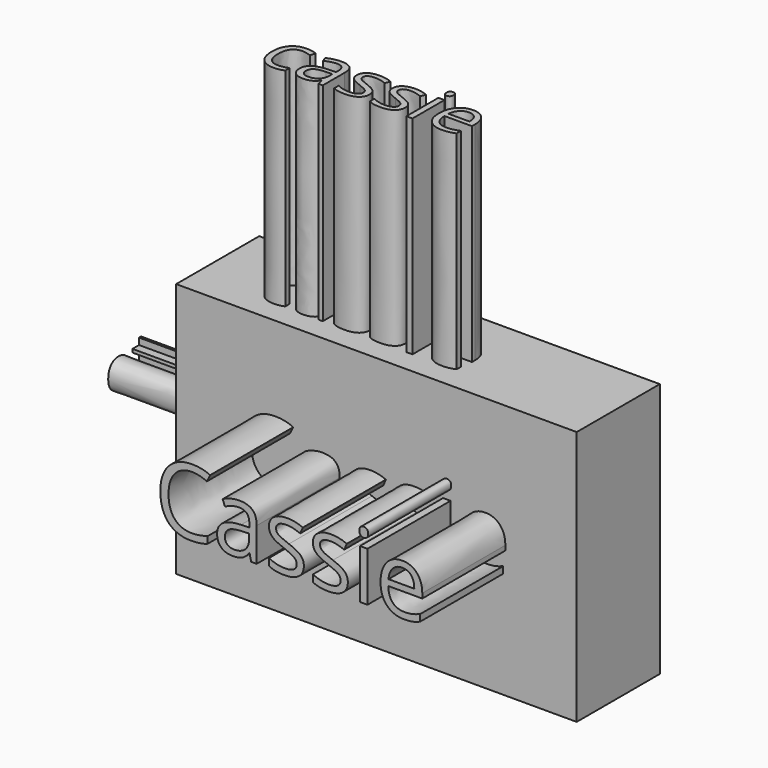
from build123d import *

# Parameters (mm, degrees)
F0_W         = 97.9832615703
F0_H         = 62.4232683331
F1_DEPTH     = 25.4
F2_TEXT_SIZE = 22.5471012527
F3_DEPTH     = 25.4
F4_TEXT_SIZE = 20.9278092834
F5_DEPTH     = 25.4
F6_TEXT_SIZE = 18.2524174711
F7_DEPTH     = 50.8
F8_TEXT_SIZE = 12.9571931514
F9_DEPTH     = 25.4


# Not quite as in the source:
# - Text() gives the source's letters only with a copy of the font that has no kerning and outlines rounded to 1/6400 em; it was checked with that copy


with BuildPart() as f1:
    # F0 (on Front) → F1 (new body)
    with BuildSketch(Plane.XZ):
        with Locations((20.3890213743, 8.9866323397)):
            Rectangle(F0_W, F0_H)
    extrude(amount=F1_DEPTH)

    # F2 (on face) → F3 (join)
    with BuildSketch(Plane.XZ.offset(25.4)):
        with Locations((-13.5282613337, 3.2854347955)):
            Text('Cassie', F2_TEXT_SIZE, font='Open Sans', text_align=(TextAlign.LEFT, TextAlign.BOTTOM))
    extrude(amount=F3_DEPTH)

    # F4 (on face) → F5 (join)
    with BuildSketch(Plane(origin=(0, 0, 0), x_dir=(-1, 0, 0), z_dir=(0, 1, 0))):
        with Locations((-20.2116858095, -5.9079082012)):
            Text('love', F4_TEXT_SIZE, font='Open Sans', text_align=(TextAlign.LEFT, TextAlign.BOTTOM))
    extrude(amount=F5_DEPTH)

    # F6 (on face) → F7 (join)
    with BuildSketch(Plane.XY.offset(40.1982665062)):
        with Locations((-14.4945653155, -19.9058707803)):
            Text('cassie', F6_TEXT_SIZE, font='Open Sans', text_align=(TextAlign.LEFT, TextAlign.BOTTOM))
    extrude(amount=F7_DEPTH)

    # F8 (on face) → F9 (join)
    with BuildSketch(Plane(origin=(-28.6026094109, 0, 0), x_dir=(0, -1, 0), z_dir=(-1, 0, 0))):
        with Locations((2.7563476469, 3.5826519597)):
            Text('to', F8_TEXT_SIZE, font='Open Sans', text_align=(TextAlign.LEFT, TextAlign.BOTTOM))
    extrude(amount=F9_DEPTH)


solid = f1.part
